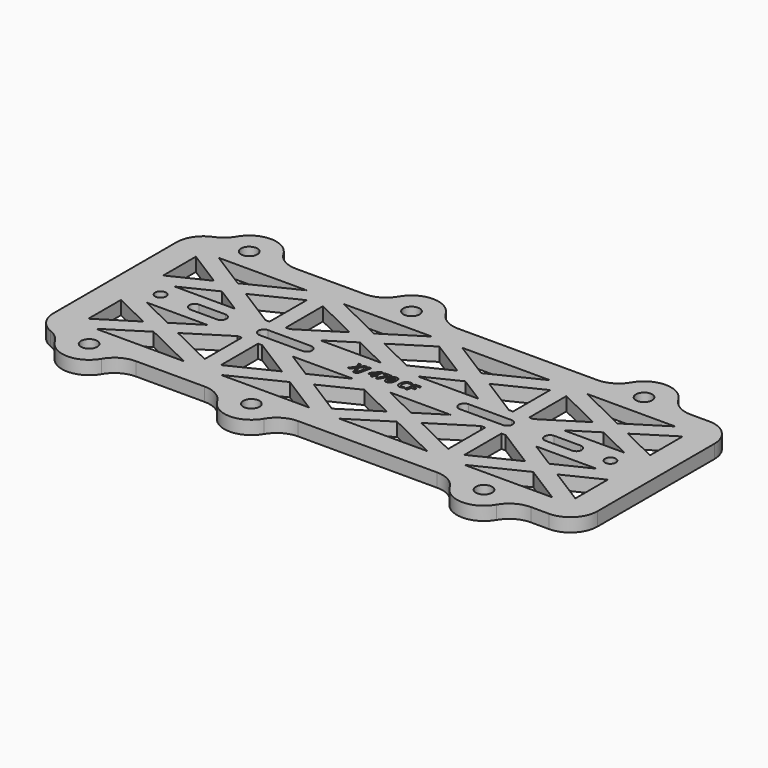
from build123d import *

# Parameters (mm, degrees)
F1_DEPTH     = 2.5
F2_R         = 5
F3_R         = 5
F4_R         = 1
F4_TEXT_SIZE = 2.7777777778
F5_DEPTH     = 2.5010001


# Not quite as in the source:
# - Text() gives the source's letters only with a copy of the font that has no kerning and outlines rounded to 1/6400 em; it was checked with that copy


with BuildPart() as f1:
    # F0 (on Top) → F1 (new body)
    with BuildSketch(Plane.XY):
        with BuildLine():
            Line((-15, 18.5), (-35, 18.5))
            ThreePointArc((-35, 18.5), (-40, 13.5), (-45, 18.5))
            Line((-45, 18.5), (-50, 18.5))
            Line((-50, 18.5), (-50, -18.5))
            Line((-50, -18.5), (-45, -18.5))
            ThreePointArc((-45, -18.5), (-40, -13.5), (-35, -18.5))
            Line((-35, -18.5), (-15, -18.5))
            ThreePointArc((-15, -18.5), (-10, -13.5), (-5, -18.5))
            Line((-5, -18.5), (28, -18.5))
            ThreePointArc((28, -18.5), (33, -13.5), (38, -18.5))
            Line((38, -18.5), (50, -18.5))
            Line((50, -18.5), (50, 18.5))
            Line((50, 18.5), (38, 18.5))
            ThreePointArc((38, 18.5), (33, 13.5), (28, 18.5))
            Line((28, 18.5), (-5, 18.5))
            ThreePointArc((-5, 18.5), (-10, 13.5), (-15, 18.5))
        make_face()
        with BuildLine():
            Line((-35, 18.5), (-38.5, 18.5))
            ThreePointArc((-38.5, 18.5), (-40, 17), (-41.5, 18.5))
            Line((-41.5, 18.5), (-45, 18.5))
            ThreePointArc((-45, 18.5), (-40, 13.5), (-35, 18.5))
        make_face()
        with BuildLine():
            ThreePointArc((-41.5, 18.5), (-40, 20), (-38.5, 18.5))
            Line((-38.5, 18.5), (-35, 18.5))
            ThreePointArc((-35, 18.5), (-40, 23.5), (-45, 18.5))
            Line((-45, 18.5), (-41.5, 18.5))
        make_face()
        with BuildLine():
            ThreePointArc((-5, 18.5), (-10, 23.5), (-15, 18.5))
            Line((-15, 18.5), (-11.5, 18.5))
            ThreePointArc((-11.5, 18.5), (-10, 20), (-8.5, 18.5))
            Line((-8.5, 18.5), (-5, 18.5))
        make_face()
        with BuildLine():
            Line((-11.5, 18.5), (-15, 18.5))
            ThreePointArc((-15, 18.5), (-10, 13.5), (-5, 18.5))
            Line((-5, 18.5), (-8.5, 18.5))
            ThreePointArc((-8.5, 18.5), (-10, 17), (-11.5, 18.5))
        make_face()
        with BuildLine():
            ThreePointArc((38, 18.5), (33, 23.5), (28, 18.5))
            Line((28, 18.5), (31.5, 18.5))
            ThreePointArc((31.5, 18.5), (33, 20), (34.5, 18.5))
            Line((34.5, 18.5), (38, 18.5))
        make_face()
        with BuildLine():
            Line((31.5, 18.5), (28, 18.5))
            ThreePointArc((28, 18.5), (33, 13.5), (38, 18.5))
            Line((38, 18.5), (34.5, 18.5))
            ThreePointArc((34.5, 18.5), (33, 17), (31.5, 18.5))
        make_face()
        with BuildLine():
            ThreePointArc((28, -18.5), (33, -23.5), (38, -18.5))
            Line((38, -18.5), (34.5, -18.5))
            ThreePointArc((34.5, -18.5), (33, -20), (31.5, -18.5))
            Line((31.5, -18.5), (28, -18.5))
        make_face()
        with BuildLine():
            Line((34.5, -18.5), (38, -18.5))
            ThreePointArc((38, -18.5), (33, -13.5), (28, -18.5))
            Line((28, -18.5), (31.5, -18.5))
            ThreePointArc((31.5, -18.5), (33, -17), (34.5, -18.5))
        make_face()
        with BuildLine():
            ThreePointArc((-5, -18.5), (-10, -13.5), (-15, -18.5))
            Line((-15, -18.5), (-11.5, -18.5))
            ThreePointArc((-11.5, -18.5), (-10, -17), (-8.5, -18.5))
            Line((-8.5, -18.5), (-5, -18.5))
        make_face()
        with BuildLine():
            Line((-11.5, -18.5), (-15, -18.5))
            ThreePointArc((-15, -18.5), (-10, -23.5), (-5, -18.5))
            Line((-5, -18.5), (-8.5, -18.5))
            ThreePointArc((-8.5, -18.5), (-10, -20), (-11.5, -18.5))
        make_face()
        with BuildLine():
            Line((-41.5, -18.5), (-45, -18.5))
            ThreePointArc((-45, -18.5), (-40, -23.5), (-35, -18.5))
            Line((-35, -18.5), (-38.5, -18.5))
            ThreePointArc((-38.5, -18.5), (-40, -20), (-41.5, -18.5))
        make_face()
        with BuildLine():
            ThreePointArc((-35, -18.5), (-40, -13.5), (-45, -18.5))
            Line((-45, -18.5), (-41.5, -18.5))
            ThreePointArc((-41.5, -18.5), (-40, -17), (-38.5, -18.5))
            Line((-38.5, -18.5), (-35, -18.5))
        make_face()
    extrude(amount=F1_DEPTH)

    # F2
    f2_edges = [f1.edges().sort_by_distance(p)[0] for p in [
        (-35, -18.5, 1.25),
        (-5, -18.5, 1.25),
        (38, -18.5, 1.25),
        (50, -18.5, 1.25),
        (50, 18.5, 1.25),
        (-45, -18.5, 1.25),
        (-15, -18.5, 1.25),
        (28, -18.5, 1.25),
        (28, 18.5, 1.25),
        (-15, 18.5, 1.25),
        (-45, 18.5, 1.25),
        (38, 18.5, 1.25),
        (-5, 18.5, 1.25),
        (-35, 18.5, 1.25),
    ]]
    fillet(f2_edges, radius=F2_R)

    # F3
    f3_edges = [f1.edges().sort_by_distance(p)[0] for p in [
        (-50, 18.5, 1.25),
        (-50, -18.5, 1.25),
    ]]
    fillet(f3_edges, radius=F3_R)

    # F4 (on face) → F5 (cut, through all)
    with BuildSketch(Plane.XY.offset(2.5)):
        Polygon((-45, 12.4204197702), (-45, 4.8765684233), (-38.2592312178, 8.16805779), align=None)
        Polygon((-25.9185698741, 14.193951409), (-42.1886291052, 14.193951409), (-35.0897714405, 9.71569182), align=None)
        Polygon((-24, 11.7922341919), (-32.1066303703, 7.8338002912), (-24.7727761987, 3.2072949689), (-24, 3.2072949689), align=None)
        Polygon((-35.2760901476, 6.2861662613), (-41.5814301259, 3.2072949689), (-30.3955179882, 3.2072949689), align=None)
        with Locations((-41.5814301259, 0)):
            Circle(F4_R)
        with BuildLine():
            Line((-35.2760901476, -1), (-30.3955179882, -1))
            ThreePointArc((-30.3955179882, -1), (-29.3955179882, 0), (-30.3955179882, 1))
            Line((-30.3955179882, 1), (-35.2760901476, 1))
            ThreePointArc((-35.2760901476, 1), (-36.2760901476, 0), (-35.2760901476, -1))
        make_face()
        with BuildLine():
            Line((-22.5, -1), (-14.55679629, -1))
            ThreePointArc((-14.55679629, -1), (-13.55679629, 0), (-14.55679629, 1))
            Line((-14.55679629, 1), (-22.5, 1))
            ThreePointArc((-22.5, 1), (-23.5, 0), (-22.5, -1))
        make_face()
        Polygon((-12.8933696297, 7.8338002912), (-21, 11.7922341919), (-21, 3.2072949689), (-20.2272238013, 3.2072949689), align=None)
        Polygon((-3.4185698741, 3.2072949689), (-9.7239098524, 6.2861662613), (-14.6044820118, 3.2072949689), align=None)
        Polygon((-3.4185698741, -3.2072949689), (-14.6044820118, -3.2072949689), (-9.7239098524, -6.2861662613), align=None)
        Polygon((-20.2272238013, -3.2072949689), (-21, -3.2072949689), (-21, -11.7922341919), (-12.8933696297, -7.8338002912), align=None)
        Polygon((-24.7727761987, -3.2072949689), (-32.1066303703, -7.8338002912), (-24, -11.7922341919), (-24, -3.2072949689), align=None)
        Polygon((-30.3955179882, -3.2072949689), (-41.5814301259, -3.2072949689), (-35.2760901476, -6.2861662613), align=None)
        Polygon((-45, -4.8765684233), (-45, -12.4204197702), (-38.2592312178, -8.16805779), align=None)
        Polygon((-35.0897714405, -9.71569182), (-42.1886291052, -14.193951409), (-25.9185698741, -14.193951409), align=None)
        Polygon((-9.9102285595, -9.71569182), (-19.0814301259, -14.193951409), (-2.8113708948, -14.193951409), align=None)
        Polygon((-6.7407687822, -8.16805779), (0, -12.4204197702), (6.7407687822, -8.16805779), (0, -4.8765684233), align=None)
        Polygon((-2.8113708948, 14.193951409), (-19.0814301259, 14.193951409), (-9.9102285595, 9.71569182), align=None)
        Polygon((6.7407687822, 8.16805779), (0, 12.4204197702), (-6.7407687822, 8.16805779), (0, 4.8765684233), align=None)
        Polygon((19.0814301259, 14.193951409), (2.8113708948, 14.193951409), (9.9102285595, 9.71569182), align=None)
        Polygon((9.7239098524, 6.2861662613), (3.4185698741, 3.2072949689), (14.6044820118, 3.2072949689), align=None)
        Polygon((21, 3.2072949689), (21, 11.7922341919), (12.8933696297, 7.8338002912), (20.2272238013, 3.2072949689), align=None)
        Polygon((32.1066303703, 7.8338002912), (24, 11.7922341919), (24, 3.2072949689), (24.7727761987, 3.2072949689), align=None)
        Polygon((42.1886291052, 14.193951409), (25.9185698741, 14.193951409), (35.0897714405, 9.71569182), align=None)
        Polygon((35.2760901476, 6.2861662613), (30.3955179882, 3.2072949689), (41.5814301259, 3.2072949689), align=None)
        Polygon((38.2592312178, 8.16805779), (45, 4.8765684233), (45, 12.4204197702), align=None)
        Polygon((41.5814301259, -3.2072949689), (30.3955179882, -3.2072949689), (35.2760901476, -6.2730461431), align=None)
        Polygon((38.2781657875, -8.1588121184), (45, -12.3811595106), (45, -4.8765684233), align=None)
        Polygon((35.0897714405, -9.71569182), (25.9185698741, -14.193951409), (42.1886291052, -14.193951409), align=None)
        Polygon((23.9907571534, -3.2072949689), (23.9907571534, -11.7601448559), (32.0889812195, -7.8226664606), (24.7727761987, -3.2072949689), align=None)
        Polygon((21, -11.7922341919), (21, -3.2072949689), (20.2272238013, -3.2072949689), (12.8933696297, -7.8338002912), align=None)
        Polygon((14.6044820118, -3.2072949689), (3.4185698741, -3.2072949689), (9.7239098524, -6.2861662613), align=None)
        Polygon((9.9102285595, -9.71569182), (2.8113708948, -14.193951409), (19.0814301259, -14.193951409), align=None)
        with BuildLine():
            Line((22.5, 1), (14.55679629, 1))
            ThreePointArc((14.55679629, 1), (13.55679629, 0), (14.55679629, -1))
            Line((14.55679629, -1), (22.5, -1))
            ThreePointArc((22.5, -1), (23.5, 0), (22.5, 1))
        make_face()
        with BuildLine():
            Line((30.3955179882, -1), (35.2760901476, -1))
            ThreePointArc((35.2760901476, -1), (36.2760901476, 0), (35.2760901476, 1))
            Line((35.2760901476, 1), (30.3955179882, 1))
            ThreePointArc((30.3955179882, 1), (29.3955179882, 0), (30.3955179882, -1))
        make_face()
        with Locations((41.5814301259, 0)):
            Circle(F4_R)
        with Locations((-6.044921875, -1)):
            Text('XJ 470 CF', F4_TEXT_SIZE, font='Open Sans', font_style=FontStyle.BOLDITALIC, text_align=(TextAlign.LEFT, TextAlign.BOTTOM))
    extrude(amount=-F5_DEPTH, mode=Mode.SUBTRACT)


solid = f1.part
